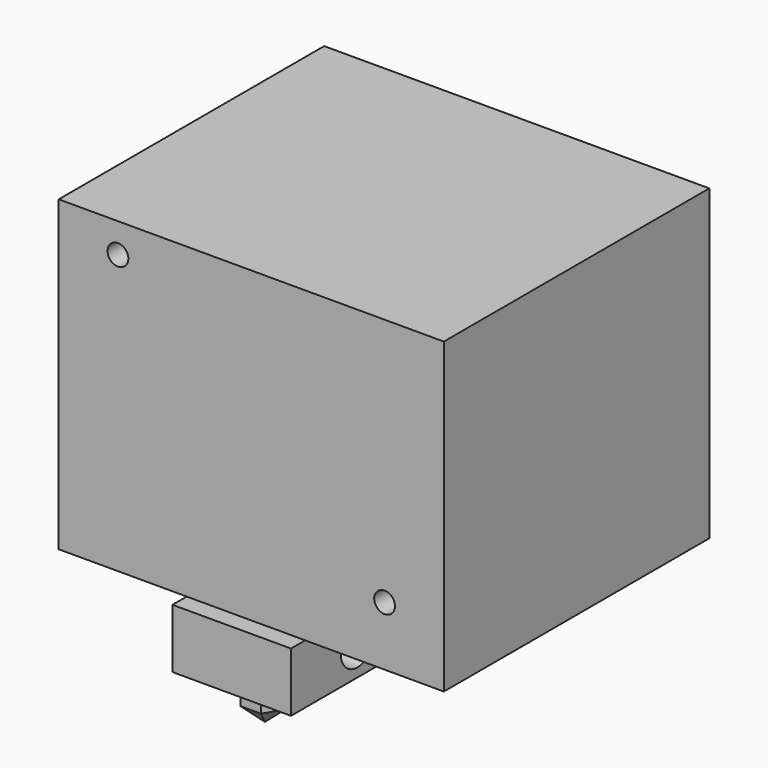
from build123d import *

# Parameters (mm, degrees)
F0_W      = 20
F0_H      = 20
F1_DEPTH  = 10
F2_R      = 3.5
F3_DEPTH  = 20.001
F4_R      = 3
F5_DEPTH  = 35
F7_DEPTH  = 4
F11_W     = 65
F11_H     = 56
F12_DEPTH = 52
F13_R     = 1.75
F14_DEPTH = 25


# Not quite as in the source:
# - an extrude whose draft closes it to a point is written as a loft to that point


with BuildPart() as f1:
    # F0 (on Top) → F1 (new body)
    with BuildSketch(Plane.XY):
        Rectangle(F0_W, F0_H)
    extrude(amount=F1_DEPTH)

    # F2 (on face) → F3 (cut, through all)
    with BuildSketch(Plane.YZ.offset(10)):
        with Locations((4, 5)):
            Circle(F2_R)
    extrude(amount=-F3_DEPTH, mode=Mode.SUBTRACT)

    # F4 (on face) → F5 (join)
    with BuildSketch(Plane.XY.offset(10)):
        with Locations((0, -3)):
            Circle(F4_R)
    extrude(amount=F5_DEPTH)

    # F6 (on face) → F7 (join)
    with BuildSketch(Plane(origin=(0, 0, 0), x_dir=(1, 0, 0), z_dir=(0, 0, -1))):
        Polygon((-3.4641016151, 3), (-1.7320508076, 0), (1.7320508076, 0), (3.4641016151, 3), (1.7320508076, 6), (-1.7320508076, 6), align=None)
    extrude(amount=F7_DEPTH)

    # F7_face (on face) → F8 section 0
    with BuildSketch(Plane(origin=(0, -3, -4), x_dir=(1, 0, 0), z_dir=(0, 0, -1)), mode=Mode.PRIVATE) as f8_s0:
        Polygon((-1.7320508076, 3), (-3.4641016151, 0), (-1.7320508076, -3), (1.7320508076, -3), (3.4641016151, 0), (1.7320508076, 3), align=None)
    loft([f8_s0.sketch, Vertex(0, -3, -7)], ruled=True)

    # F11 (on offset) → F12 (join)
    with BuildSketch(Plane.XY.offset(28)):
        with Locations((22.5, -6)):
            Rectangle(F11_W, F11_H)
    extrude(amount=F12_DEPTH)

    # F13 (on face) → F14 (cut)
    with BuildSketch(Plane.XZ.offset(34)):
        with Locations((0, 75)):
            Circle(F13_R)
        with Locations((45, 38)):
            Circle(F13_R)
    extrude(amount=-F14_DEPTH, mode=Mode.SUBTRACT)


solid = f1.part
